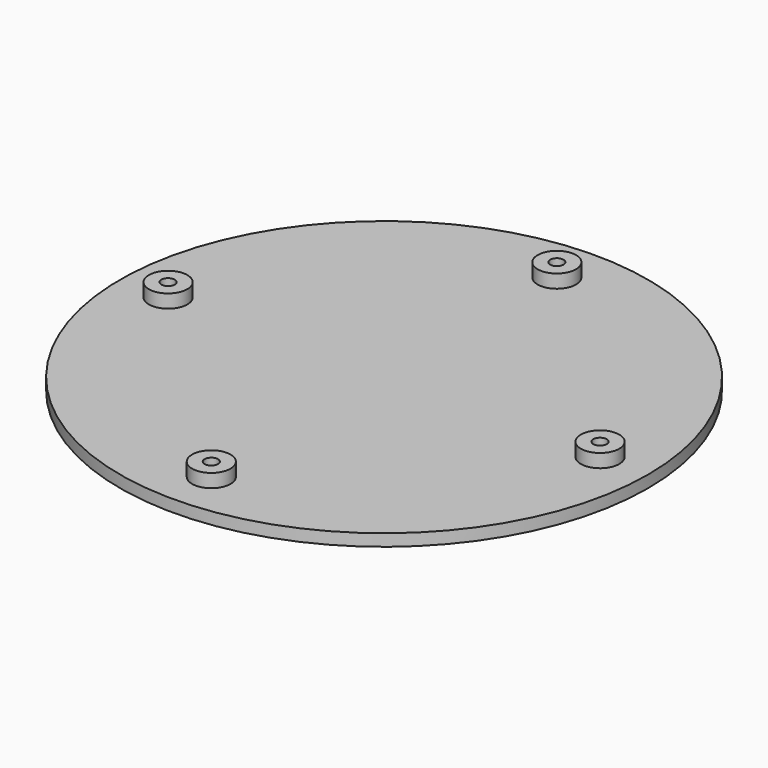
from build123d import *

# Parameters (mm, degrees)
F0_R     = 55
F1_DEPTH = 2.5
F2_R     = 1.4
F3_DEPTH = 12.5
F2_R_2   = 4
F4_DEPTH = 5.3


with BuildPart() as f1:
    # F0 (on Top) → F1 (new body)
    with BuildSketch(Plane.XY):
        Circle(F0_R)
    extrude(amount=F1_DEPTH)

    # F2 (on face) → F3 (cut, symmetric)
    with BuildSketch(Plane(origin=(0, 0, 0), x_dir=(1, 0, 0), z_dir=(0, 0, -1))):
        with Locations((0, -45)):
            Circle(F2_R)
        with Locations((-45, 0)):
            Circle(F2_R)
        with Locations((0, 45)):
            Circle(F2_R)
        with Locations((45, 0)):
            Circle(F2_R)
    extrude(amount=F3_DEPTH, both=True, mode=Mode.SUBTRACT)

    # F2 (on face) → F4 (join)
    with BuildSketch(Plane(origin=(0, 0, 0), x_dir=(1, 0, 0), z_dir=(0, 0, -1))):
        with Locations((-45, 0)):
            Circle(F2_R_2)
        with Locations((-45, 0)):
            Circle(F2_R, mode=Mode.SUBTRACT)
        with Locations((0, -45)):
            Circle(F2_R_2)
        with Locations((0, -45)):
            Circle(F2_R, mode=Mode.SUBTRACT)
        with Locations((45, 0)):
            Circle(F2_R_2)
        with Locations((45, 0)):
            Circle(F2_R, mode=Mode.SUBTRACT)
        with Locations((0, 45)):
            Circle(F2_R_2)
        with Locations((0, 45)):
            Circle(F2_R, mode=Mode.SUBTRACT)
    extrude(amount=-F4_DEPTH)


solid = f1.part
